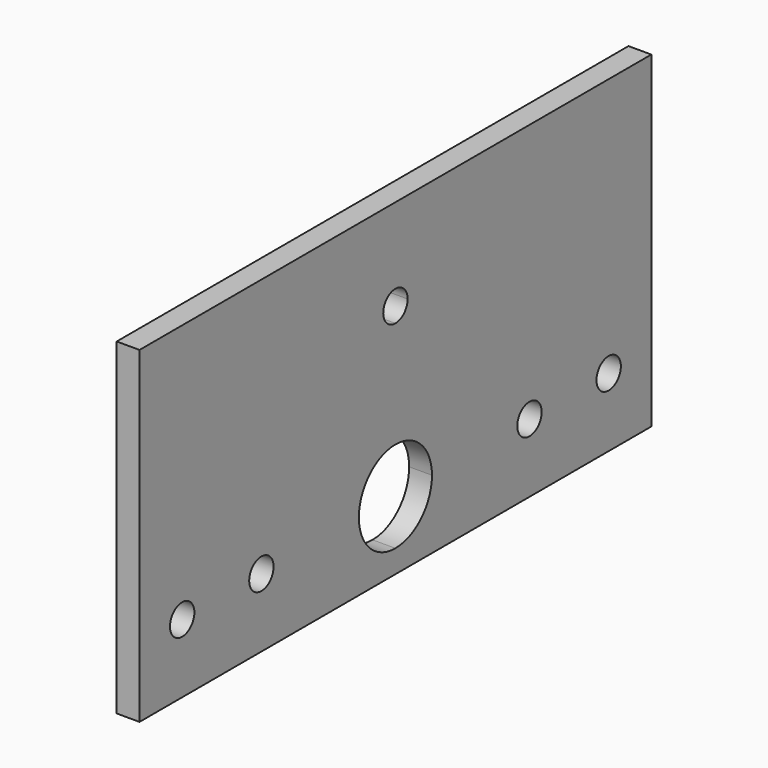
from build123d import *

# Parameters (mm, degrees)
F1_DEPTH = 3


with BuildPart() as f1:
    # F0 (on Right) → F1 (new body)
    with BuildSketch(Plane.YZ):
        with BuildLine():
            Line((-33, 9), (-33, 0))
            Line((-33, 0), (-24, 0))
            ThreePointArc((-24, 0), (-26.6360389693, 6.3639610307), (-33, 9))
        make_face()
        with BuildLine():
            ThreePointArc((-37, 0), (-35, 2), (-33, 0))
            Line((-33, 0), (-33, 9))
            ThreePointArc((-33, 9), (-39.3639610307, 6.3639610307), (-42, 0))
            Line((-42, 0), (-37, 0))
        make_face()
        with BuildLine():
            Line((-24, 0), (-33, 0))
            Line((-33, 0), (-33, -9))
            ThreePointArc((-33, -9), (-26.6360389693, -6.3639610307), (-24, 0))
        make_face()
        with BuildLine():
            Line((-33, -9), (-33, 0))
            ThreePointArc((-33, 0), (-35, -2), (-37, 0))
            Line((-37, 0), (-42, 0))
            ThreePointArc((-42, 0), (-39.3639610307, -6.3639610307), (-33, -9))
        make_face()
        with BuildLine():
            ThreePointArc((-20, 0), (-22, -2), (-24, 0))
            ThreePointArc((-24, 0), (-26.6360389693, -6.3639610307), (-33, -9))
            Line((-33, -9), (-25, -9))
            Line((-25, -9), (-4.3588989435, -9))
            ThreePointArc((-4.3588989435, -9), (-8.4731632061, -5.310885546), (-10, 0))
            Line((-10, 0), (-20, 0))
        make_face()
        with BuildLine():
            ThreePointArc((-33, 9), (-26.6360389693, 6.3639610307), (-24, 0))
            ThreePointArc((-24, 0), (-22, 2), (-20, 0))
            Line((-20, 0), (-10, 0))
            ThreePointArc((-10, 0), (-7.0710678119, 7.0710678119), (0, 10))
            Line((0, 10), (0, 20))
            ThreePointArc((0, 20), (-2, 21.9999999928), (-1.44e-08, 24))
            ThreePointArc((-1.44e-08, 24), (-4.7434164964, 25.3514707334), (-8.0622577483, 29))
            Line((-8.0622577483, 29), (-9, 29))
            Line((-9, 29), (-9, 25))
            ThreePointArc((-9, 25), (-13.686291501, 13.686291501), (-25, 9))
            Line((-25, 9), (-33, 9))
        make_face()
        with BuildLine():
            ThreePointArc((-42, 0), (-39.3639610307, 6.3639610307), (-33, 9))
            Line((-33, 9), (-25, 9))
            ThreePointArc((-25, 9), (-13.686291501, 13.686291501), (-9, 25))
            Line((-9, 25), (-9, 29))
            Line((-9, 29), (-42, 29))
            Line((-42, 29), (-42, 0))
        make_face()
        with BuildLine():
            Line((-42, -9), (-33, -9))
            ThreePointArc((-33, -9), (-39.3639610307, -6.3639610307), (-42, 0))
            Line((-42, 0), (-42, -9))
        make_face()
        with BuildLine():
            ThreePointArc((0, 10), (-7.0710678119, 7.0710678119), (-10, 0))
            Line((-10, 0), (-6, 0))
            ThreePointArc((-6, 0), (-4.2426406871, 4.2426406871), (0, 6))
            Line((0, 6), (0, 10))
        make_face()
        with BuildLine():
            Line((-6, 0), (-10, 0))
            ThreePointArc((-10, 0), (-8.4731632061, -5.310885546), (-4.3588989435, -9))
            Line((-4.3588989435, -9), (0, -9))
            Line((0, -9), (0, -6))
            ThreePointArc((0, -6), (-4.2426406871, -4.2426406871), (-6, 0))
        make_face()
        with BuildLine():
            Line((-42, 34), (-42, 29))
            Line((-42, 29), (-9, 29))
            Line((-9, 29), (-9, 33))
            ThreePointArc((-9, 33), (-8.9860571774, 33.5007758031), (-8.94427191, 34))
            Line((-8.94427191, 34), (-42, 34))
        make_face()
        with BuildLine():
            ThreePointArc((10, 0), (7.0710678119, 7.0710678119), (0, 10))
            Line((0, 10), (0, 6))
            ThreePointArc((0, 6), (4.2426406871, 4.2426406871), (6, 0))
            Line((6, 0), (10, 0))
        make_face()
        with BuildLine():
            Line((0, 20), (0, 10))
            ThreePointArc((0, 10), (7.0710678119, 7.0710678119), (10, 0))
            Line((10, 0), (20, 0))
            ThreePointArc((20, 0), (22, 2), (24, 0))
            ThreePointArc((24, 0), (26.6360389693, 6.3639610307), (33, 9))
            Line((33, 9), (25, 9))
            ThreePointArc((25, 9), (13.686291501, 13.686291501), (9, 25))
            Line((9, 25), (9, 29))
            Line((9, 29), (8.0622577483, 29))
            ThreePointArc((8.0622577483, 29), (4.7434164841, 25.3514707258), (-1.44e-08, 24))
            ThreePointArc((-1.44e-08, 24), (1.4142135573, 23.4142135675), (2, 22))
            ThreePointArc((2, 22), (1.4142135624, 20.5857864376), (0, 20))
        make_face()
        with BuildLine():
            Line((-9, 33), (-9, 29))
            Line((-9, 29), (-8.0622577483, 29))
            ThreePointArc((-8.0622577483, 29), (-8.7624288794, 30.9457750531), (-9, 33))
        make_face()
        with BuildLine():
            Line((0, -6), (0, -9))
            Line((0, -9), (4.3588989435, -9))
            ThreePointArc((4.3588989435, -9), (8.4731632061, -5.310885546), (10, 0))
            Line((10, 0), (6, 0))
            ThreePointArc((6, 0), (4.2426406871, -4.2426406871), (0, -6))
        make_face()
        with BuildLine():
            Line((20, 0), (10, 0))
            ThreePointArc((10, 0), (8.4731632061, -5.310885546), (4.3588989435, -9))
            Line((4.3588989435, -9), (25, -9))
            Line((25, -9), (33, -9))
            ThreePointArc((33, -9), (26.6360389693, -6.3639610307), (24, 0))
            ThreePointArc((24, 0), (22, -2), (20, 0))
        make_face()
        with BuildLine():
            Line((0, 33), (-9, 33))
            ThreePointArc((-9, 33), (-8.7624288794, 30.9457750531), (-8.0622577483, 29))
            Line((-8.0622577483, 29), (0, 29))
            Line((0, 29), (0, 33))
        make_face()
        with BuildLine():
            ThreePointArc((-8.94427191, 34), (-8.9860571774, 33.5007758031), (-9, 33))
            Line((-9, 33), (0, 33))
            ThreePointArc((0, 33), (-1, 33.2679491924), (-1.7320508076, 34))
            Line((-1.7320508076, 34), (-8.94427191, 34))
        make_face()
        with BuildLine():
            Line((0, 29), (-8.0622577483, 29))
            ThreePointArc((-8.0622577483, 29), (-4.7434164964, 25.3514707334), (-1.44e-08, 24))
            Line((0, 24), (0, 29))
        make_face()
        with BuildLine():
            Line((0, 29), (0, 24))
            ThreePointArc((-1.44e-08, 24), (4.7434164841, 25.3514707258), (8.0622577483, 29))
            Line((8.0622577483, 29), (0, 29))
        make_face()
        with BuildLine():
            ThreePointArc((-1.7320508076, 34), (-1, 33.2679491924), (0, 33))
            Line((0, 33), (0, 34))
            Line((0, 34), (-1.7320508076, 34))
        make_face()
        with BuildLine():
            ThreePointArc((1.7320508076, 34), (1, 33.2679491924), (0, 33))
            Line((0, 33), (0, 29))
            Line((0, 29), (8.0622577483, 29))
            ThreePointArc((8.0622577483, 29), (8.7624288794, 30.9457750531), (9, 33))
            ThreePointArc((9, 33), (8.9860571774, 33.5007758031), (8.94427191, 34))
            Line((8.94427191, 34), (1.7320508076, 34))
        make_face()
        with BuildLine():
            Line((0, 34), (0, 33))
            ThreePointArc((0, 33), (1, 33.2679491924), (1.7320508076, 34))
            Line((1.7320508076, 34), (0, 34))
        make_face()
        with BuildLine():
            ThreePointArc((9, 33), (8.7624288794, 30.9457750531), (8.0622577483, 29))
            Line((8.0622577483, 29), (9, 29))
            Line((9, 29), (9, 33))
        make_face()
        with BuildLine():
            ThreePointArc((33, 9), (26.6360389693, 6.3639610307), (24, 0))
            Line((24, 0), (33, 0))
            ThreePointArc((33, 0), (35, 2), (37, 0))
            Line((37, 0), (42, 0))
            ThreePointArc((42, 0), (39.3639610307, 6.3639610307), (33, 9))
        make_face()
        with BuildLine():
            Line((33, 0), (24, 0))
            ThreePointArc((24, 0), (26.6360389693, -6.3639610307), (33, -9))
            Line((33, -9), (33, 0))
        make_face()
        with BuildLine():
            Line((42, 34), (8.94427191, 34))
            ThreePointArc((8.94427191, 34), (8.9860571774, 33.5007758031), (9, 33))
            Line((9, 33), (9, 29))
            Line((9, 29), (42, 29))
            Line((42, 29), (42, 34))
        make_face()
        with BuildLine():
            Line((33, 0), (33, -9))
            ThreePointArc((33, -9), (39.3639610307, -6.3639610307), (42, 0))
            Line((42, 0), (37, 0))
            ThreePointArc((37, 0), (35, -2), (33, 0))
        make_face()
        with BuildLine():
            ThreePointArc((42, 0), (39.3639610307, -6.3639610307), (33, -9))
            Line((33, -9), (42, -9))
            Line((42, -9), (42, 0))
        make_face()
        with BuildLine():
            Line((42, 29), (9, 29))
            Line((9, 29), (9, 25))
            ThreePointArc((9, 25), (13.686291501, 13.686291501), (25, 9))
            Line((25, 9), (33, 9))
            ThreePointArc((33, 9), (39.3639610307, 6.3639610307), (42, 0))
            Line((42, 0), (42, 29))
        make_face()
    extrude(amount=F1_DEPTH)


solid = f1.part
